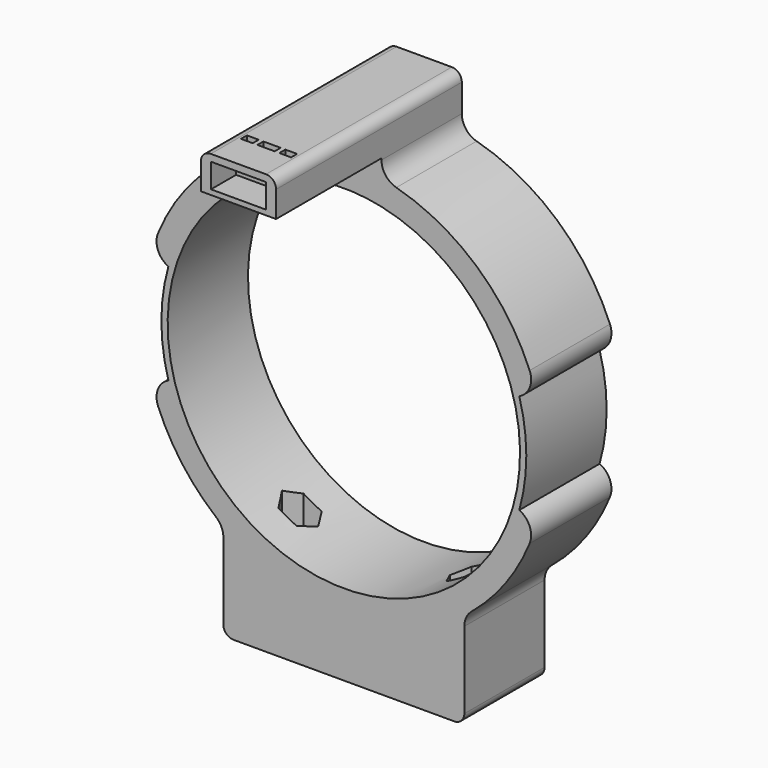
from build123d import *

# Parameters (mm, degrees)
F1_DEPTH     = 25.4
F3_DEPTH     = 6.35
F5_DEPTH     = 25.4
F6_W         = 15.08125
F6_H         = 12.7
F7_DEPTH     = 5.3578125
F8_R         = 2.5796875
F9_DEPTH     = 25.4
F12_DEPTH    = 25.4
F13_W        = 19.05
F13_H        = 9.1559581755
F14_DEPTH    = 33.3375
F15_W        = 13.890625
F15_H        = 6.1515625
F16_DEPTH    = 7.9375
F17_W        = 12.7
F17_H        = 1.905
F18_DEPTH    = 6.604
F19_W        = 1.190625
F19_H        = 1.905
F20_DEPTH    = 6.604
F21_W        = 25.003125
F21_H        = 9.921875
F22_DEPTH    = 4.5640625
F24_DEPTH    = 27.94
F25_T1_DEPTH = 59.9739709134
F26_R        = 2.54
F27_R        = 2.54
F28_R        = 5.08


# Not quite as in the source:
# - a fillet or chamfer that OpenCascade refuses, or shapes differently, is made with other operations: its cross-section is extruded or revolved along the edge and cut away or added


with BuildPart() as f1:
    # F0 (on Front) → F1 (new body)
    with BuildSketch(Plane.XZ):
        with BuildLine():
            ThreePointArc((9.525, 43.5474833257), (34.7253859158, 27.9509660298), (44.577, 0))
            ThreePointArc((44.577, 0), (-27.9509660298, -34.7253859158), (-9.525, 43.5474833257))
            Line((-9.525, 43.5474833257), (-9.525, 49.8990418245))
            ThreePointArc((-9.525, 49.8990418245), (-32.3787739113, -39.1440289189), (50.8, 0))
            ThreePointArc((50.8, 0), (39.1440289189, 32.3787739113), (9.525, 49.8990418245))
            Line((9.525, 49.8990418245), (9.525, 43.5474833257))
        make_face()
        with BuildLine():
            ThreePointArc((-9.525, 43.5474833257), (0, 44.577), (9.525, 43.5474833257))
            Line((9.525, 43.5474833257), (9.525, 49.8990418245))
            ThreePointArc((9.525, 49.8990418245), (0, 50.8), (-9.525, 49.8990418245))
            Line((-9.525, 49.8990418245), (-9.525, 43.5474833257))
        make_face()
        with BuildLine():
            ThreePointArc((-9.525, 49.8990418245), (0, 50.8), (9.525, 49.8990418245))
            Line((9.525, 49.8990418245), (9.525, 63.5))
            Line((9.525, 63.5), (-9.525, 63.5))
            Line((-9.525, 63.5), (-9.525, 49.8990418245))
        make_face()
    extrude(amount=F1_DEPTH)

    # F2 (on face) → F3 (cut)
    with BuildSketch(Plane.XZ.offset(25.4)):
        with BuildLine():
            ThreePointArc((0.8929687032, 50.3226047716), (2.6789062266, 50.322604731), (3.571875, 51.8692719891))
            ThreePointArc((3.571875, 51.8692719891), (1.7859375, 53.6552094891), (0, 51.8692719891))
            ThreePointArc((0, 51.8692719891), (0.2392702419, 50.9763032626), (0.8929687032, 50.3226047716))
        make_face()
        with BuildLine():
            ThreePointArc((-0.8929687383, 50.3226047513), (-0.2392702521, 50.976303245), (0, 51.8692719891))
            ThreePointArc((0, 51.8692719891), (-3.3326047479, 52.7622407333), (-0.8929687383, 50.3226047513))
        make_face()
        with BuildLine():
            ThreePointArc((0.8929687032, 50.3226047716), (0.2392702419, 50.9763032626), (0, 51.8692719891))
            ThreePointArc((0, 51.8692719891), (-0.2392702521, 50.976303245), (-0.8929687383, 50.3226047513))
            ThreePointArc((-0.8929687383, 50.3226047513), (-2.03e-08, 50.561875), (0.8929687032, 50.3226047716))
        make_face()
        with BuildLine():
            ThreePointArc((1.7859375, 48.7759375), (1.546667231, 49.6689062734), (0.8929687032, 50.3226047716))
            ThreePointArc((0.8929687032, 50.3226047716), (-2.03e-08, 50.561875), (-0.8929687383, 50.3226047513))
            ThreePointArc((-0.8929687383, 50.3226047513), (-0.8929687558, 47.2292702588), (1.7859375, 48.7759375))
        make_face()
    extrude(amount=-F3_DEPTH, mode=Mode.SUBTRACT)

    # F4 (on Front) → F5 (join)
    with BuildSketch(Plane.XZ):
        with BuildLine():
            Line((-30.48, -65.0875), (30.48, -65.0875))
            Line((30.48, -65.0875), (30.48, -40.64))
            ThreePointArc((30.48, -40.64), (0, -50.8), (-30.48, -40.64))
            Line((-30.48, -40.64), (-30.48, -65.0875))
        make_face()
    extrude(amount=F5_DEPTH)

    # F6 (on face) → F7 (cut)
    with BuildSketch(Plane(origin=(0, 0, -65.0875), x_dir=(1, 0, 0), z_dir=(0, 0, -1))):
        with Locations((20.0421875, 12.7)):
            Rectangle(F6_W, F6_H)
        with Locations((-20.0421875, 12.7)):
            Rectangle(F6_W, F6_H)
    extrude(amount=-F7_DEPTH, mode=Mode.SUBTRACT)

    # F8 (on face) → F9 (cut)
    with BuildSketch(Plane(origin=(0, 0, -59.7296875), x_dir=(1, 0, 0), z_dir=(0, 0, -1))):
        with Locations((21.2328125, 12.7)):
            Circle(F8_R)
        with Locations((-21.2328125, 12.7)):
            Circle(F8_R)
    extrude(amount=-F9_DEPTH, mode=Mode.SUBTRACT)

    # F11 (on offset) → F12 (cut)
    with BuildSketch(Plane.XY.offset(-48.26)):
        Polygon((18.9414536192, -16.66875), (23.5241713808, -16.66875), (25.8155302617, -12.7), (23.5241713808, -8.73125), (18.9414536192, -8.73125), (16.6500947383, -12.7), align=None)
        Polygon((-25.8155302617, -12.7), (-23.5241713808, -16.66875), (-18.9414536192, -16.66875), (-16.6500947383, -12.7), (-18.9414536192, -8.73125), (-23.5241713808, -8.73125), align=None)
    extrude(amount=F12_DEPTH, mode=Mode.SUBTRACT)

    # F13 (on face) → F14 (join)
    with BuildSketch(Plane.XZ.offset(25.4)):
        with Locations((0, 58.9220209122)):
            Rectangle(F13_W, F13_H)
    extrude(amount=F14_DEPTH)

    # F15 (on face) → F16 (cut)
    with BuildSketch(Plane.XZ.offset(58.7375)):
        with Locations((0, 58.6898230745)):
            Rectangle(F15_W, F15_H)
    extrude(amount=-F16_DEPTH, mode=Mode.SUBTRACT)

    # F17 (on face) → F18 (cut)
    with BuildSketch(Plane.XY.offset(63.5)):
        with Locations((0, -49.05375)):
            Rectangle(F17_W, F17_H)
    extrude(amount=-F18_DEPTH, mode=Mode.SUBTRACT)

    # F19 (on face) → F20 (join)
    with BuildSketch(Plane.XY.offset(56.896)):
        with Locations((-2.778125, -49.05375)):
            Rectangle(F19_W, F19_H)
        with Locations((2.778125, -49.05375)):
            Rectangle(F19_W, F19_H)
    extrude(amount=F20_DEPTH)

    # F21 (on face) → F22 (cut)
    with BuildSketch(Plane(origin=(0, 0, -65.0875), x_dir=(1, 0, 0), z_dir=(0, 0, -1))):
        with Locations((0, 12.7)):
            Rectangle(F21_W, F21_H)
    extrude(amount=-F22_DEPTH, mode=Mode.SUBTRACT)

    # F23 (on face) → F24 (cut)
    with BuildSketch(Plane.XZ.offset(25.4)):
        with BuildLine():
            ThreePointArc((44.3832294932, 12.7), (46.1645, 0), (44.3832294932, -12.7))
            Line((44.3832294932, -12.7), (55.8275170624, -12.7))
            Line((55.8275170624, -12.7), (55.8275170624, 12.7))
            Line((55.8275170624, 12.7), (44.3832294932, 12.7))
        make_face()
        with BuildLine():
            Line((-44.3832294932, 12.7), (-55.6385964155, 12.7))
            Line((-55.6385964155, 12.7), (-55.6385964155, -12.7))
            Line((-55.6385964155, -12.7), (-44.3832294932, -12.7))
            ThreePointArc((-44.3832294932, -12.7), (-46.1645, 0), (-44.3832294932, 12.7))
        make_face()
    extrude(amount=-F24_DEPTH, mode=Mode.SUBTRACT)

    # F25: fillet of radius 5.08 on 4 edges, made by hand

    # F25_s2 → F25_t1 (cut)
    with BuildSketch(Plane.XZ.offset(-17.2869854567)):
        with BuildLine():
            ThreePointArc((-44.3832294932, 12.7), (-47.0229133194, 15.4501150062), (-47.0065282778, 19.2620429672))
            Line((-47.0065282778, 19.2620429672), (-47.1005413343, 19.3005670532))
            ThreePointArc((-47.1005413343, 19.3005670532), (-48.3049064769, 16.050199152), (-49.2852622738, 12.7254))
            Line((-49.2852622738, 12.7254), (-49.1868884968, 12.5984))
            ThreePointArc((-49.1868884968, 12.5984), (-46.785058995, 12.5984), (-44.4247765741, 12.6072832266))
            Line((-44.4247765741, 12.6072832266), (-44.3832294932, 12.7))
        make_face()
        with BuildLine():
            ThreePointArc((-47.0065282778, -19.2620429672), (-47.0229133194, -15.4501150062), (-44.3832294932, -12.7))
            Line((-44.3832294932, -12.7), (-44.4247765741, -12.6072832266))
            ThreePointArc((-44.4247765741, -12.6072832266), (-46.785058995, -12.5984), (-49.1868884968, -12.5984))
            Line((-49.1868884968, -12.5984), (-49.2852622738, -12.7254))
            ThreePointArc((-49.2852622738, -12.7254), (-48.3049064769, -16.050199152), (-47.1005413343, -19.3005670532))
            Line((-47.1005413343, -19.3005670532), (-47.0065282778, -19.2620429672))
        make_face()
        with BuildLine():
            ThreePointArc((44.3832294932, -12.7), (47.0229133194, -15.4501150062), (47.0065282778, -19.2620429672))
            Line((47.0065282778, -19.2620429672), (47.1005413343, -19.3005670532))
            ThreePointArc((47.1005413343, -19.3005670532), (48.3049064769, -16.050199152), (49.2852622738, -12.7254))
            Line((49.2852622738, -12.7254), (49.1868884968, -12.5984))
            ThreePointArc((49.1868884968, -12.5984), (46.785058995, -12.5984), (44.4247765741, -12.6072832266))
            Line((44.4247765741, -12.6072832266), (44.3832294932, -12.7))
        make_face()
        with BuildLine():
            ThreePointArc((47.0065282778, 19.2620429672), (47.0229133194, 15.4501150062), (44.3832294932, 12.7))
            Line((44.3832294932, 12.7), (44.4247765741, 12.6072832266))
            ThreePointArc((44.4247765741, 12.6072832266), (46.785058995, 12.5984), (49.1868884968, 12.5984))
            Line((49.1868884968, 12.5984), (49.2852622738, 12.7254))
            ThreePointArc((49.2852622738, 12.7254), (48.3049064769, 16.050199152), (47.1005413343, 19.3005670532))
            Line((47.1005413343, 19.3005670532), (47.0065282778, 19.2620429672))
        make_face()
    extrude(amount=F25_T1_DEPTH, mode=Mode.SUBTRACT)

    # F26
    f26_edges = [f1.edges().sort_by_distance(p)[0] for p in [
        (30.48, -12.7, -65.0875),
        (-30.48, -12.7, -65.0875),
    ]]
    fillet(f26_edges, radius=F26_R)

    # F27
    f27_edges = [f1.edges().sort_by_distance(p)[0] for p in [
        (9.525, -29.36875, 63.5),
        (-9.525, -29.36875, 63.5),
    ]]
    fillet(f27_edges, radius=F27_R)

    # F28
    f28_edges = [f1.edges().sort_by_distance(p)[0] for p in [
        (30.48, -12.7, -40.64),
        (-30.48, -12.7, -40.64),
        (-9.525, -12.7, 49.899042),
        (9.525, -12.7, 49.899042),
    ]]
    fillet(f28_edges, radius=F28_R)


solid = f1.part
